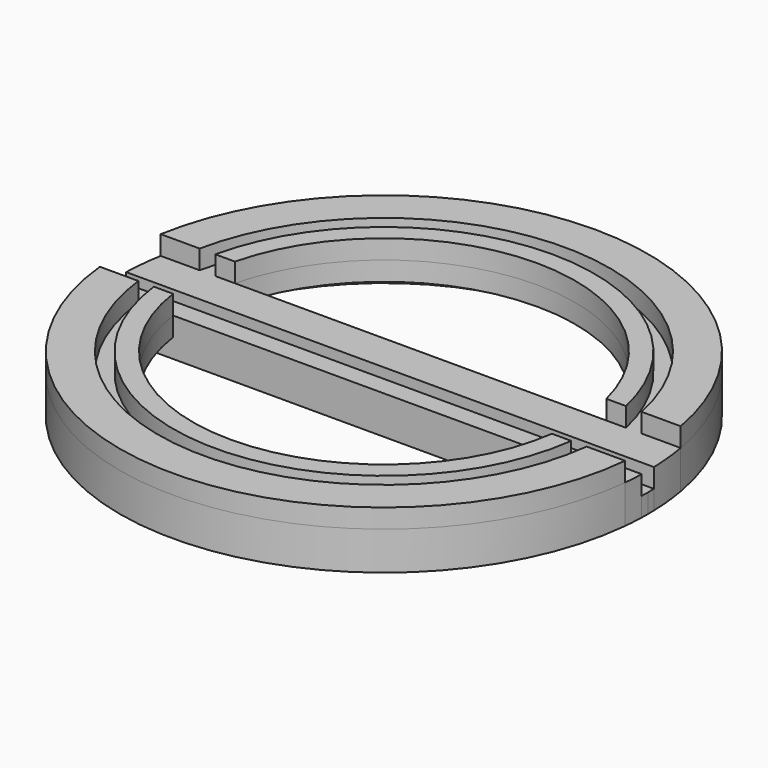
from build123d import *

# Parameters (mm, degrees)
F1_START = -5
F1_DEPTH = 5
F2_DEPTH = 5
F3_DEPTH = 10
F4_DEPTH = 5
F5_DEPTH = 5


# Not quite as in the source:
# - after a boolean that leaves OpenCascade's solid faulty, fix() repairs it
# - a feature names something its author has since deleted; it is built from what else it names


with BuildPart() as f1:
    # F0 (on Top) → F1 (new body)
    with BuildSketch(Plane.XY.offset(F1_START)):
        with BuildLine():
            Line((0, 12), (-48.538644398, 12))
            Line((-48.538644398, 12), (-53.6749476013, 12))
            Line((-53.6749476013, 12), (-57.7667724561, 12))
            Line((-57.7667724561, 12), (-67.9485099174, 12))
            ThreePointArc((-67.9485099174, 12), (-68.6421053306, 7.0186448683), (-68.9710084021, 2))
            Line((-68.9710084021, 2), (0, 2))
            Line((0, 2), (0, 12))
        make_face()
        with BuildLine():
            Line((0, -7), (0, -2))
            Line((0, -2), (-68.9710084021, -2))
            ThreePointArc((-68.9710084021, -2), (-68.8529103806, -4.5029692558), (-68.6440092069, -7))
            Line((-68.6440092069, -7), (-58.5832740635, -7))
            Line((-58.5832740635, -7), (-54.5527267879, -7))
            Line((-54.5527267879, -7), (-49.5075751779, -7))
            Line((-49.5075751779, -7), (0, -7))
        make_face()
        with BuildLine():
            Line((68.9710084021, -2), (0, -2))
            Line((0, -2), (0, -7))
            Line((0, -7), (49.5075751779, -7))
            Line((49.5075751779, -7), (54.5527267879, -7))
            Line((54.5527267879, -7), (58.5832740635, -7))
            Line((58.5832740635, -7), (68.6440092069, -7))
            ThreePointArc((68.6440092069, -7), (68.8529103806, -4.5029692558), (68.9710084021, -2))
        make_face()
        with BuildLine():
            Line((68.9710084021, 2), (0, 2))
            Line((0, 2), (0, 0))
            Line((0, 0), (0, -2))
            Line((0, -2), (68.9710084021, -2))
            ThreePointArc((68.9710084021, -2), (68.9927517198, -1.0001050586), (69, 0))
            ThreePointArc((69, 0), (68.9927517198, 1.0001050586), (68.9710084021, 2))
        make_face()
        with BuildLine():
            Line((53.6749476013, 12), (48.538644398, 12))
            Line((48.538644398, 12), (0, 12))
            Line((0, 12), (0, 2))
            Line((0, 2), (68.9710084021, 2))
            ThreePointArc((68.9710084021, 2), (68.6421053306, 7.0186448683), (67.9485099174, 12))
            Line((67.9485099174, 12), (57.7667724561, 12))
            Line((57.7667724561, 12), (53.6749476013, 12))
        make_face()
        with BuildLine():
            Line((0, 0), (0, 2))
            Line((0, 2), (-68.9710084021, 2))
            ThreePointArc((-68.9710084021, 2), (-69, 0), (-68.9710084021, -2))
            Line((-68.9710084021, -2), (0, -2))
            Line((0, -2), (0, 0))
        make_face()
    extrude(amount=-F1_DEPTH)

    # F0 (on Top) → F2 (join)
    with BuildSketch(Plane.XY):
        with BuildLine():
            Line((0, -7), (0, -2))
            Line((0, -2), (-68.9710084021, -2))
            ThreePointArc((-68.9710084021, -2), (-68.8529103806, -4.5029692558), (-68.6440092069, -7))
            Line((-68.6440092069, -7), (-58.5832740635, -7))
            Line((-58.5832740635, -7), (-54.5527267879, -7))
            Line((-54.5527267879, -7), (-49.5075751779, -7))
            Line((-49.5075751779, -7), (0, -7))
        make_face()
        with BuildLine():
            Line((0, 12), (-48.538644398, 12))
            Line((-48.538644398, 12), (-53.6749476013, 12))
            Line((-53.6749476013, 12), (-57.7667724561, 12))
            Line((-57.7667724561, 12), (-67.9485099174, 12))
            ThreePointArc((-67.9485099174, 12), (-68.6421053306, 7.0186448683), (-68.9710084021, 2))
            Line((-68.9710084021, 2), (0, 2))
            Line((0, 2), (0, 12))
        make_face()
        with BuildLine():
            Line((53.6749476013, 12), (48.538644398, 12))
            Line((48.538644398, 12), (0, 12))
            Line((0, 12), (0, 2))
            Line((0, 2), (68.9710084021, 2))
            ThreePointArc((68.9710084021, 2), (68.6421053306, 7.0186448683), (67.9485099174, 12))
            Line((67.9485099174, 12), (57.7667724561, 12))
            Line((57.7667724561, 12), (53.6749476013, 12))
        make_face()
        with BuildLine():
            Line((68.9710084021, -2), (0, -2))
            Line((0, -2), (0, -7))
            Line((0, -7), (49.5075751779, -7))
            Line((49.5075751779, -7), (54.5527267879, -7))
            Line((54.5527267879, -7), (58.5832740635, -7))
            Line((58.5832740635, -7), (68.6440092069, -7))
            ThreePointArc((68.6440092069, -7), (68.8529103806, -4.5029692558), (68.9710084021, -2))
        make_face()
    extrude(amount=-F2_DEPTH)

    # F0 (on Top) → F3 (join)
    with BuildSketch(Plane.XY):
        with BuildLine():
            ThreePointArc((-57.7667724561, 12), (0, 59), (57.7667724561, 12))
            Line((57.7667724561, 12), (67.9485099174, 12))
            ThreePointArc((67.9485099174, 12), (0, 69), (-67.9485099174, 12))
            Line((-67.9485099174, 12), (-57.7667724561, 12))
        make_face()
        with BuildLine():
            Line((-58.5832740635, -7), (-68.6440092069, -7))
            ThreePointArc((-68.6440092069, -7), (0, -69), (68.6440092069, -7))
            Line((68.6440092069, -7), (58.5832740635, -7))
            ThreePointArc((58.5832740635, -7), (0, -59), (-58.5832740635, -7))
        make_face()
    extrude(amount=-F3_DEPTH)

    # F0 (on Top) → F4 (join)
    with BuildSketch(Plane.XY):
        with BuildLine():
            Line((54.5527267879, -7), (49.5075751779, -7))
            ThreePointArc((49.5075751779, -7), (0, -50), (-49.5075751779, -7))
            Line((-49.5075751779, -7), (-54.5527267879, -7))
            ThreePointArc((-54.5527267879, -7), (0, -55), (54.5527267879, -7))
        make_face()
        with BuildLine():
            ThreePointArc((-48.538644398, 12), (0, 50), (48.538644398, 12))
            Line((48.538644398, 12), (53.6749476013, 12))
            ThreePointArc((53.6749476013, 12), (0, 55), (-53.6749476013, 12))
            Line((-53.6749476013, 12), (-48.538644398, 12))
        make_face()
        with BuildLine():
            ThreePointArc((-53.6749476013, 12), (0, 55), (53.6749476013, 12))
            Line((53.6749476013, 12), (57.7667724561, 12))
            ThreePointArc((57.7667724561, 12), (0, 59), (-57.7667724561, 12))
            Line((-57.7667724561, 12), (-53.6749476013, 12))
        make_face()
        with BuildLine():
            Line((-54.5527267879, -7), (-58.5832740635, -7))
            ThreePointArc((-58.5832740635, -7), (0, -59), (58.5832740635, -7))
            Line((58.5832740635, -7), (54.5527267879, -7))
            ThreePointArc((54.5527267879, -7), (0, -55), (-54.5527267879, -7))
        make_face()
    extrude(amount=-F4_DEPTH)

    # F0 (on Top) → F5 (join)
    with BuildSketch(Plane.XY):
        with BuildLine():
            ThreePointArc((-57.7667724561, 12), (0, 59), (57.7667724561, 12))
            Line((57.7667724561, 12), (67.9485099174, 12))
            ThreePointArc((67.9485099174, 12), (0, 69), (-67.9485099174, 12))
            Line((-67.9485099174, 12), (-57.7667724561, 12))
        make_face()
        with BuildLine():
            ThreePointArc((-48.538644398, 12), (0, 50), (48.538644398, 12))
            Line((48.538644398, 12), (53.6749476013, 12))
            ThreePointArc((53.6749476013, 12), (0, 55), (-53.6749476013, 12))
            Line((-53.6749476013, 12), (-48.538644398, 12))
        make_face()
        with BuildLine():
            Line((-58.5832740635, -7), (-68.6440092069, -7))
            ThreePointArc((-68.6440092069, -7), (0, -69), (68.6440092069, -7))
            Line((68.6440092069, -7), (58.5832740635, -7))
            ThreePointArc((58.5832740635, -7), (0, -59), (-58.5832740635, -7))
        make_face()
        with BuildLine():
            Line((54.5527267879, -7), (49.5075751779, -7))
            ThreePointArc((49.5075751779, -7), (0, -50), (-49.5075751779, -7))
            Line((-49.5075751779, -7), (-54.5527267879, -7))
            ThreePointArc((-54.5527267879, -7), (0, -55), (54.5527267879, -7))
        make_face()
    extrude(amount=F5_DEPTH)

    add(f1.part.fix(), mode=Mode.REPLACE)


solid = f1.part
